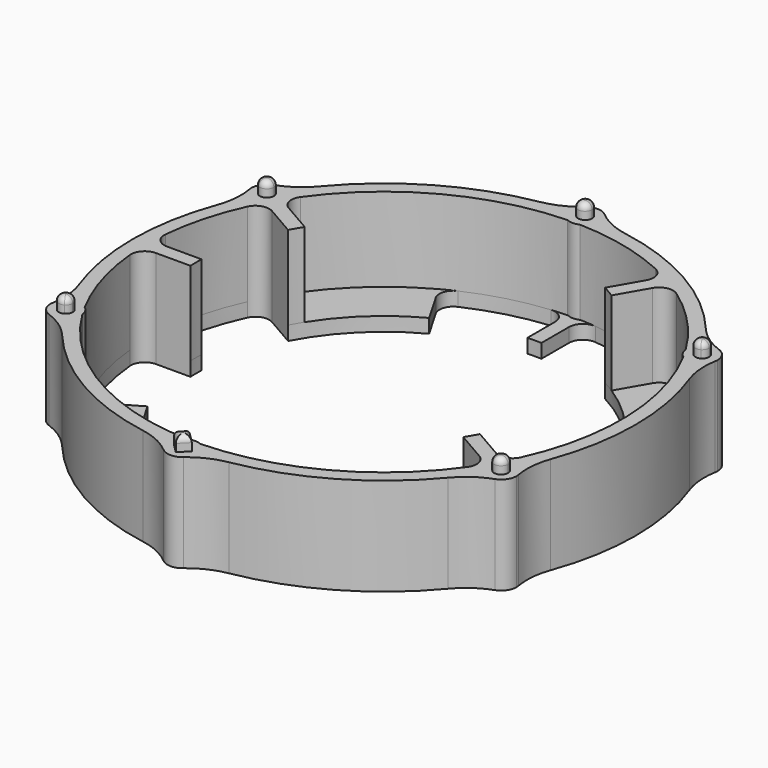
from build123d import *

# Parameters (mm, degrees)
F1_R         = 18
F1_R_2       = 17
F2_DEPTH     = 7
F3_DEPTH     = 7
F4_DEPTH     = 1
F6_DEPTH     = 7
F7_R         = 1
F8_R         = 5
F9_DEPTH     = 8
F10_R        = 0.44999
F11_DEPTH    = 1.8
F12_R        = 13.47
F13_DEPTH    = 1
F14_DEPTH    = 1
F15_T1_DEPTH = 3.7395798703
F15_T3_DEPTH = 1


# Not quite as in the source:
# - a fillet or chamfer that OpenCascade refuses, or shapes differently, is made with other operations: its cross-section is extruded or revolved along the edge and cut away or added
# - a fillet or chamfer is up to 0.001 mm smaller than in the source, because OpenCascade refuses the exact size


with BuildPart() as f2:
    # F1 (on Top) → F2 (new body)
    with BuildSketch(Plane.XY):
        Circle(F1_R)
        Circle(F1_R_2, mode=Mode.SUBTRACT)
    extrude(amount=F2_DEPTH)

    # F0 (on Top) → F3 (join)
    with BuildSketch(Plane.XY):
        with BuildLine():
            Line((-11.4073228059, 7.1633711619), (-14.4660626528, 8.9293354359))
            ThreePointArc((-14.4660626528, 8.9293354359), (-14.7224318643, 8.5), (-14.9660626528, 8.0633100321))
            Line((-14.9660626528, 8.0633100321), (-11.9073228059, 6.2973457581))
            ThreePointArc((-11.9073228059, 6.2973457581), (-11.665362189, 6.735), (-11.4073228059, 7.1633711619))
        make_face()
        with BuildLine():
            Line((7.1633711619, 11.4073228059), (8.9293354359, 14.4660626528))
            ThreePointArc((8.9293354359, 14.4660626528), (8.5, 14.7224318643), (8.0633100321, 14.9660626528))
            Line((8.0633100321, 14.9660626528), (6.2973457581, 11.9073228059))
            ThreePointArc((6.2973457581, 11.9073228059), (6.735, 11.665362189), (7.1633711619, 11.4073228059))
        make_face()
        with BuildLine():
            ThreePointArc((14.4660626528, -8.9293354359), (14.7224318643, -8.5), (14.9660626528, -8.0633100321))
            Line((14.9660626528, -8.0633100321), (11.9073228059, -6.2973457581))
            ThreePointArc((11.9073228059, -6.2973457581), (11.665362189, -6.735), (11.4073228059, -7.1633711619))
            Line((11.4073228059, -7.1633711619), (14.4660626528, -8.9293354359))
        make_face()
        with BuildLine():
            Line((-13.46071692, 0.5), (-16.992645468, 0.5))
            ThreePointArc((-16.992645468, 0.5), (-17, 0), (-16.992645468, -0.5))
            Line((-16.992645468, -0.5), (-13.46071692, -0.5))
            ThreePointArc((-13.46071692, -0.5), (-13.47, 0), (-13.46071692, 0.5))
        make_face()
    extrude(amount=F3_DEPTH)

    # F1 (on Top) → F4 (join)
    with BuildSketch(Plane.XY):
        Circle(F1_R)
        Circle(F1_R_2, mode=Mode.SUBTRACT)
        Circle(F1_R_2)
    extrude(amount=F4_DEPTH)

    # F5 (on Top) → F6 (join)
    with BuildSketch(Plane.XY):
        with BuildLine():
            ThreePointArc((-14.4884572681, 9), (-14.6275367743, 9.5353800561), (-15.0096060035, 9.935377578))
            ThreePointArc((-15.0096060035, 9.935377578), (-15.1731450826, 9.6837837802), (-15.3324673166, 9.4294987133))
            ThreePointArc((-15.3324673166, 9.4294987133), (-15.153718855, 9.2469868663), (-15.0884572681, 9))
            ThreePointArc((-15.0884572681, 9), (-15.3354561915, 8.5687338928), (-15.832419089, 8.5635568422))
            ThreePointArc((-15.832419089, 8.5635568422), (-15.9729752997, 8.2984372068), (-16.1090923805, 8.0310113108))
            ThreePointArc((-16.1090923805, 8.0310113108), (-15.0239657375, 8.0558870238), (-14.4884572681, 9))
        make_face()
        with BuildLine():
            ThreePointArc((-15.3324673166, 9.4294987133), (-15.1731450826, 9.6837837802), (-15.0096060035, 9.935377578))
            ThreePointArc((-15.0096060035, 9.935377578), (-16.5410852123, 9.55), (-16.1090923805, 8.0310113108))
            ThreePointArc((-16.1090923805, 8.0310113108), (-15.9729752997, 8.2984372068), (-15.832419089, 8.5635568422))
            ThreePointArc((-15.832419089, 8.5635568422), (-16.02146997, 9.25), (-15.3324673166, 9.4294987133))
        make_face()
        with BuildLine():
            ThreePointArc((-1.099486377, 17.9663888889), (0, 16.9), (1.099486377, 17.9663888889))
            ThreePointArc((1.099486377, 17.9663888889), (0.7998302171, 17.982220987), (0.4999517724, 17.9930555556))
            ThreePointArc((0.4999517724, 17.9930555556), (0, 17.5), (-0.4999517724, 17.9930555556))
            ThreePointArc((-0.4999517724, 17.9930555556), (-0.7998302171, 17.982220987), (-1.099486377, 17.9663888889))
        make_face()
        with BuildLine():
            ThreePointArc((0.4999517724, 17.9930555556), (0.7998302171, 17.982220987), (1.099486377, 17.9663888889))
            ThreePointArc((1.099486377, 17.9663888889), (1.0998715868, 17.9831924823), (1.1, 18))
            ThreePointArc((1.1, 18), (-0.0168075177, 19.0998715868), (-1.099486377, 17.9663888889))
            ThreePointArc((-1.099486377, 17.9663888889), (-0.7998302171, 17.982220987), (-0.4999517724, 17.9930555556))
            ThreePointArc((-0.4999517724, 17.9930555556), (-0.003472306, 18.4999879429), (0.5, 18))
            ThreePointArc((0.5, 18), (0.4999879429, 17.996527694), (0.4999517724, 17.9930555556))
        make_face()
        with BuildLine():
            ThreePointArc((15.832419089, 8.5635568422), (15.9729752997, 8.2984372068), (16.1090923805, 8.0310113108))
            ThreePointArc((16.1090923805, 8.0310113108), (16.5325702443, 8.4355084694), (16.6884572681, 9))
            ThreePointArc((16.6884572681, 9), (16.1238373242, 9.9609204939), (15.0096060035, 9.935377578))
            ThreePointArc((15.0096060035, 9.935377578), (15.1731450826, 9.6837837802), (15.3324673166, 9.4294987133))
            ThreePointArc((15.3324673166, 9.4294987133), (15.8354441344, 9.4347384132), (16.0884572681, 9))
            ThreePointArc((16.0884572681, 9), (16.0197233753, 8.7469989234), (15.832419089, 8.5635568422))
        make_face()
        with BuildLine():
            ThreePointArc((15.0096060035, 9.935377578), (14.635829324, 8.45), (16.1090923805, 8.0310113108))
            ThreePointArc((16.1090923805, 8.0310113108), (15.9729752997, 8.2984372068), (15.832419089, 8.5635568422))
            ThreePointArc((15.832419089, 8.5635568422), (15.1554445662, 8.75), (15.3324673166, 9.4294987133))
            ThreePointArc((15.3324673166, 9.4294987133), (15.1731450826, 9.6837837802), (15.0096060035, 9.935377578))
        make_face()
        with BuildLine():
            ThreePointArc((-15.3324673166, -9.4294987133), (-15.1731450826, -9.6837837802), (-15.0096060035, -9.935377578))
            ThreePointArc((-15.0096060035, -9.935377578), (-14.6275367743, -9.5353800561), (-14.4884572681, -9))
            ThreePointArc((-14.4884572681, -9), (-15.0239657375, -8.0558870238), (-16.1090923805, -8.0310113108))
            ThreePointArc((-16.1090923805, -8.0310113108), (-15.9729752997, -8.2984372068), (-15.832419089, -8.5635568422))
            ThreePointArc((-15.832419089, -8.5635568422), (-15.3354561915, -8.5687338928), (-15.0884572681, -9))
            ThreePointArc((-15.0884572681, -9), (-15.153718855, -9.2469868663), (-15.3324673166, -9.4294987133))
        make_face()
        with BuildLine():
            ThreePointArc((-16.1090923805, -8.0310113108), (-16.5410852123, -9.55), (-15.0096060035, -9.935377578))
            ThreePointArc((-15.0096060035, -9.935377578), (-15.1731450826, -9.6837837802), (-15.3324673166, -9.4294987133))
            ThreePointArc((-15.3324673166, -9.4294987133), (-16.02146997, -9.25), (-15.832419089, -8.5635568422))
            ThreePointArc((-15.832419089, -8.5635568422), (-15.9729752997, -8.2984372068), (-16.1090923805, -8.0310113108))
        make_face()
        with BuildLine():
            ThreePointArc((0.6255239257, -17.9891278226), (0.8625800837, -17.9793202207), (1.099486377, -17.9663888889))
            ThreePointArc((1.099486377, -17.9663888889), (0, -16.9), (-1.099486377, -17.9663888889))
            ThreePointArc((-1.099486377, -17.9663888889), (-0.8625800837, -17.9793202207), (-0.6255239257, -17.9891278226))
            Line((-0.6255239257, -17.9891278226), (0, -17.3636038969))
            Line((0, -17.3636038969), (0.6255239257, -17.9891278226))
        make_face()
        with BuildLine():
            ThreePointArc((1.1, -18), (1.0998715868, -17.9831924823), (1.099486377, -17.9663888889))
            ThreePointArc((1.099486377, -17.9663888889), (0.8625800837, -17.9793202207), (0.6255239257, -17.9891278226))
            Line((0.6255239257, -17.9891278226), (0.6363961031, -18))
            Line((0.6363961031, -18), (0, -18.6363961031))
            Line((0, -18.6363961031), (-0.6363961031, -18))
            Line((-0.6363961031, -18), (-0.6255239257, -17.9891278226))
            ThreePointArc((-0.6255239257, -17.9891278226), (-0.8625800837, -17.9793202207), (-1.099486377, -17.9663888889))
            ThreePointArc((-1.099486377, -17.9663888889), (-0.0168075177, -19.0998715868), (1.1, -18))
        make_face()
        with BuildLine():
            ThreePointArc((16.6884572681, -9), (16.5325702443, -8.4355084694), (16.1090923805, -8.0310113108))
            ThreePointArc((16.1090923805, -8.0310113108), (15.9729752997, -8.2984372068), (15.832419089, -8.5635568422))
            ThreePointArc((15.832419089, -8.5635568422), (16.0197233753, -8.7469989234), (16.0884572681, -9))
            ThreePointArc((16.0884572681, -9), (15.8354441344, -9.4347384132), (15.3324673166, -9.4294987133))
            ThreePointArc((15.3324673166, -9.4294987133), (15.1731450826, -9.6837837802), (15.0096060035, -9.935377578))
            ThreePointArc((15.0096060035, -9.935377578), (16.1238373242, -9.9609204939), (16.6884572681, -9))
        make_face()
        with BuildLine():
            ThreePointArc((15.832419089, -8.5635568422), (15.9729752997, -8.2984372068), (16.1090923805, -8.0310113108))
            ThreePointArc((16.1090923805, -8.0310113108), (14.635829324, -8.45), (15.0096060035, -9.935377578))
            ThreePointArc((15.0096060035, -9.935377578), (15.1731450826, -9.6837837802), (15.3324673166, -9.4294987133))
            ThreePointArc((15.3324673166, -9.4294987133), (15.1554445662, -8.75), (15.832419089, -8.5635568422))
        make_face()
        with BuildLine():
            ThreePointArc((-15.0884572681, 9), (-15.153718855, 9.2469868663), (-15.3324673166, 9.4294987133))
            ThreePointArc((-15.3324673166, 9.4294987133), (-15.5884572681, 9), (-15.832419089, 8.5635568422))
            ThreePointArc((-15.832419089, 8.5635568422), (-15.3354561915, 8.5687338928), (-15.0884572681, 9))
        make_face()
        with BuildLine():
            ThreePointArc((-15.832419089, 8.5635568422), (-15.5884572681, 9), (-15.3324673166, 9.4294987133))
            ThreePointArc((-15.3324673166, 9.4294987133), (-16.02146997, 9.25), (-15.832419089, 8.5635568422))
        make_face()
        with BuildLine():
            ThreePointArc((-0.4999517724, 17.9930555556), (0, 18), (0.4999517724, 17.9930555556))
            ThreePointArc((0.4999517724, 17.9930555556), (0.4999879429, 17.996527694), (0.5, 18))
            ThreePointArc((0.5, 18), (-0.003472306, 18.4999879429), (-0.4999517724, 17.9930555556))
        make_face()
        with BuildLine():
            ThreePointArc((-0.4999517724, 17.9930555556), (0, 17.5), (0.4999517724, 17.9930555556))
            ThreePointArc((0.4999517724, 17.9930555556), (0, 18), (-0.4999517724, 17.9930555556))
        make_face()
        with BuildLine():
            ThreePointArc((15.3324673166, 9.4294987133), (15.5884572681, 9), (15.832419089, 8.5635568422))
            ThreePointArc((15.832419089, 8.5635568422), (16.0197233753, 8.7469989234), (16.0884572681, 9))
            ThreePointArc((16.0884572681, 9), (15.8354441344, 9.4347384132), (15.3324673166, 9.4294987133))
        make_face()
        with BuildLine():
            ThreePointArc((15.3324673166, 9.4294987133), (15.1554445662, 8.75), (15.832419089, 8.5635568422))
            ThreePointArc((15.832419089, 8.5635568422), (15.5884572681, 9), (15.3324673166, 9.4294987133))
        make_face()
        with BuildLine():
            ThreePointArc((16.0884572681, -9), (16.0197233753, -8.7469989234), (15.832419089, -8.5635568422))
            ThreePointArc((15.832419089, -8.5635568422), (15.5884572681, -9), (15.3324673166, -9.4294987133))
            ThreePointArc((15.3324673166, -9.4294987133), (15.8354441344, -9.4347384132), (16.0884572681, -9))
        make_face()
        with BuildLine():
            ThreePointArc((15.3324673166, -9.4294987133), (15.5884572681, -9), (15.832419089, -8.5635568422))
            ThreePointArc((15.832419089, -8.5635568422), (15.1554445662, -8.75), (15.3324673166, -9.4294987133))
        make_face()
        with BuildLine():
            Line((0.6363961031, -18), (0.6255239257, -17.9891278226))
            ThreePointArc((0.6255239257, -17.9891278226), (0, -18), (-0.6255239257, -17.9891278226))
            Line((-0.6255239257, -17.9891278226), (-0.6363961031, -18))
            Line((-0.6363961031, -18), (0, -18.6363961031))
            Line((0, -18.6363961031), (0.6363961031, -18))
        make_face()
        with BuildLine():
            ThreePointArc((-15.832419089, -8.5635568422), (-16.02146997, -9.25), (-15.3324673166, -9.4294987133))
            ThreePointArc((-15.3324673166, -9.4294987133), (-15.5884572681, -9), (-15.832419089, -8.5635568422))
        make_face()
        with BuildLine():
            ThreePointArc((-15.832419089, -8.5635568422), (-15.5884572681, -9), (-15.3324673166, -9.4294987133))
            ThreePointArc((-15.3324673166, -9.4294987133), (-15.153718855, -9.2469868663), (-15.0884572681, -9))
            ThreePointArc((-15.0884572681, -9), (-15.3354561915, -8.5687338928), (-15.832419089, -8.5635568422))
        make_face()
        with BuildLine():
            ThreePointArc((-0.6255239257, -17.9891278226), (0, -18), (0.6255239257, -17.9891278226))
            Line((0.6255239257, -17.9891278226), (0, -17.3636038969))
            Line((0, -17.3636038969), (-0.6255239257, -17.9891278226))
        make_face()
    extrude(amount=F6_DEPTH)

    # F7
    f7_edges = [f2.edges().sort_by_distance(p)[0] for p in [
        (8.06331, 14.966063, 4),
        (-16.992645, 0.5, 4),
        (14.966063, -8.06331, 4),
        (-16.992645, -0.5, 4),
        (-14.966063, 8.06331, 4),
        (-14.466063, 8.929335, 4),
        (8.929335, 14.466063, 4),
        (14.466063, -8.929335, 4),
    ]]
    fillet(f7_edges, radius=F7_R)

    # F8 (call 1 of 12: OpenCascade refuses the feature's edges together)
    f8_edges = [f2.edges().sort_by_distance(p)[0] for p in [
        (-16.109092, 8.031011, 3.5),
    ]]
    fillet(f8_edges, radius=F8_R)

    # F8#2 (call 2 of 12)
    f8_2_edges = [f2.edges().sort_by_distance(p)[0] for p in [
        (-15.009606, 9.935378, 3.5),
    ]]
    fillet(f8_2_edges, radius=F8_R)

    # F8#3 (call 3 of 12)
    f8_3_edges = [f2.edges().sort_by_distance(p)[0] for p in [
        (-1.099486, 17.966389, 3.5),
    ]]
    fillet(f8_3_edges, radius=F8_R)

    # F8#4 (call 4 of 12)
    f8_4_edges = [f2.edges().sort_by_distance(p)[0] for p in [
        (1.099486, 17.966389, 3.5),
    ]]
    fillet(f8_4_edges, radius=F8_R)

    # F8#5 (call 5 of 12)
    f8_5_edges = [f2.edges().sort_by_distance(p)[0] for p in [
        (-15.009606, -9.935378, 3.5),
    ]]
    fillet(f8_5_edges, radius=F8_R)

    # F8#6 (call 6 of 12)
    f8_6_edges = [f2.edges().sort_by_distance(p)[0] for p in [
        (-16.109092, -8.031011, 3.5),
    ]]
    fillet(f8_6_edges, radius=F8_R)

    # F8#7 (call 7 of 12)
    f8_7_edges = [f2.edges().sort_by_distance(p)[0] for p in [
        (1.099486, -17.966389, 3.5),
    ]]
    fillet(f8_7_edges, radius=F8_R)

    # F8#8 (call 8 of 12)
    f8_8_edges = [f2.edges().sort_by_distance(p)[0] for p in [
        (-1.099486, -17.966389, 3.5),
    ]]
    fillet(f8_8_edges, radius=F8_R)

    # F8#10 (call 9 of 12)
    f8_10_edges = [f2.edges().sort_by_distance(p)[0] for p in [
        (15.009606, -9.935378, 3.5),
    ]]
    fillet(f8_10_edges, radius=F8_R)

    # F8#11 (call 10 of 12)
    f8_11_edges = [f2.edges().sort_by_distance(p)[0] for p in [
        (16.109092, 8.031011, 3.5),
    ]]
    fillet(f8_11_edges, radius=F8_R)

    # F8#12 (call 11 of 12)
    f8_12_edges = [f2.edges().sort_by_distance(p)[0] for p in [
        (15.009606, 9.935378, 3.5),
    ]]
    fillet(f8_12_edges, radius=F8_R)

    # F8#9 (call 12 of 12)
    f8_9_edges = [f2.edges().sort_by_distance(p)[0] for p in [
        (16.109092, -8.031011, 3.5),
    ]]
    fillet(f8_9_edges, radius=F8_R)

    # F5 (on Top) → F9 (join)
    with BuildSketch(Plane.XY):
        with BuildLine():
            ThreePointArc((-15.832419089, 8.5635568422), (-15.5884572681, 9), (-15.3324673166, 9.4294987133))
            ThreePointArc((-15.3324673166, 9.4294987133), (-16.02146997, 9.25), (-15.832419089, 8.5635568422))
        make_face()
        with BuildLine():
            ThreePointArc((-15.0884572681, 9), (-15.153718855, 9.2469868663), (-15.3324673166, 9.4294987133))
            ThreePointArc((-15.3324673166, 9.4294987133), (-15.5884572681, 9), (-15.832419089, 8.5635568422))
            ThreePointArc((-15.832419089, 8.5635568422), (-15.3354561915, 8.5687338928), (-15.0884572681, 9))
        make_face()
        with BuildLine():
            ThreePointArc((-0.4999517724, 17.9930555556), (0, 18), (0.4999517724, 17.9930555556))
            ThreePointArc((0.4999517724, 17.9930555556), (0.4999879429, 17.996527694), (0.5, 18))
            ThreePointArc((0.5, 18), (-0.003472306, 18.4999879429), (-0.4999517724, 17.9930555556))
        make_face()
        with BuildLine():
            ThreePointArc((-0.4999517724, 17.9930555556), (0, 17.5), (0.4999517724, 17.9930555556))
            ThreePointArc((0.4999517724, 17.9930555556), (0, 18), (-0.4999517724, 17.9930555556))
        make_face()
        with BuildLine():
            ThreePointArc((15.3324673166, 9.4294987133), (15.1554445662, 8.75), (15.832419089, 8.5635568422))
            ThreePointArc((15.832419089, 8.5635568422), (15.5884572681, 9), (15.3324673166, 9.4294987133))
        make_face()
        with BuildLine():
            ThreePointArc((15.3324673166, 9.4294987133), (15.5884572681, 9), (15.832419089, 8.5635568422))
            ThreePointArc((15.832419089, 8.5635568422), (16.0197233753, 8.7469989234), (16.0884572681, 9))
            ThreePointArc((16.0884572681, 9), (15.8354441344, 9.4347384132), (15.3324673166, 9.4294987133))
        make_face()
        with BuildLine():
            ThreePointArc((15.3324673166, -9.4294987133), (15.5884572681, -9), (15.832419089, -8.5635568422))
            ThreePointArc((15.832419089, -8.5635568422), (15.1554445662, -8.75), (15.3324673166, -9.4294987133))
        make_face()
        with BuildLine():
            ThreePointArc((16.0884572681, -9), (16.0197233753, -8.7469989234), (15.832419089, -8.5635568422))
            ThreePointArc((15.832419089, -8.5635568422), (15.5884572681, -9), (15.3324673166, -9.4294987133))
            ThreePointArc((15.3324673166, -9.4294987133), (15.8354441344, -9.4347384132), (16.0884572681, -9))
        make_face()
        with BuildLine():
            Line((0.6363961031, -18), (0.6255239257, -17.9891278226))
            ThreePointArc((0.6255239257, -17.9891278226), (0, -18), (-0.6255239257, -17.9891278226))
            Line((-0.6255239257, -17.9891278226), (-0.6363961031, -18))
            Line((-0.6363961031, -18), (0, -18.6363961031))
            Line((0, -18.6363961031), (0.6363961031, -18))
        make_face()
        with BuildLine():
            ThreePointArc((-0.6255239257, -17.9891278226), (0, -18), (0.6255239257, -17.9891278226))
            Line((0.6255239257, -17.9891278226), (0, -17.3636038969))
            Line((0, -17.3636038969), (-0.6255239257, -17.9891278226))
        make_face()
        with BuildLine():
            ThreePointArc((-15.832419089, -8.5635568422), (-16.02146997, -9.25), (-15.3324673166, -9.4294987133))
            ThreePointArc((-15.3324673166, -9.4294987133), (-15.5884572681, -9), (-15.832419089, -8.5635568422))
        make_face()
        with BuildLine():
            ThreePointArc((-15.832419089, -8.5635568422), (-15.5884572681, -9), (-15.3324673166, -9.4294987133))
            ThreePointArc((-15.3324673166, -9.4294987133), (-15.153718855, -9.2469868663), (-15.0884572681, -9))
            ThreePointArc((-15.0884572681, -9), (-15.3354561915, -8.5687338928), (-15.832419089, -8.5635568422))
        make_face()
    extrude(amount=F9_DEPTH)

    # F10 (radius 0.45 in the source; OpenCascade refuses exactly that, so slightly less here)
    f10_edges = [f2.edges().sort_by_distance(p)[0] for p in [
        (-15.844447, -8.570501, 8),
        (-15.344495, 9.436443, 8),
        (0.499952, 18.006944, 8),
        (15.344495, 9.436443, 8),
        (15.844447, -8.570501, 8),
        (0.318198, -17.681802, 8),
        (-0.318198, -18.318198, 8),
        (0.318198, -18.318198, 8),
        (-0.318198, -17.681802, 8),
    ]]
    fillet(f10_edges, radius=F10_R)

    # F5 (on Top) → F11 (cut)
    with BuildSketch(Plane.XY):
        with BuildLine():
            ThreePointArc((-15.832419089, -8.5635568422), (-16.02146997, -9.25), (-15.3324673166, -9.4294987133))
            ThreePointArc((-15.3324673166, -9.4294987133), (-15.5884572681, -9), (-15.832419089, -8.5635568422))
        make_face()
        with BuildLine():
            ThreePointArc((-15.832419089, -8.5635568422), (-15.5884572681, -9), (-15.3324673166, -9.4294987133))
            ThreePointArc((-15.3324673166, -9.4294987133), (-15.153718855, -9.2469868663), (-15.0884572681, -9))
            ThreePointArc((-15.0884572681, -9), (-15.3354561915, -8.5687338928), (-15.832419089, -8.5635568422))
        make_face()
        with BuildLine():
            Line((0.6363961031, -18), (0.6255239257, -17.9891278226))
            ThreePointArc((0.6255239257, -17.9891278226), (0, -18), (-0.6255239257, -17.9891278226))
            Line((-0.6255239257, -17.9891278226), (-0.6363961031, -18))
            Line((-0.6363961031, -18), (0, -18.6363961031))
            Line((0, -18.6363961031), (0.6363961031, -18))
        make_face()
        with BuildLine():
            ThreePointArc((-0.6255239257, -17.9891278226), (0, -18), (0.6255239257, -17.9891278226))
            Line((0.6255239257, -17.9891278226), (0, -17.3636038969))
            Line((0, -17.3636038969), (-0.6255239257, -17.9891278226))
        make_face()
        with BuildLine():
            ThreePointArc((15.3324673166, -9.4294987133), (15.5884572681, -9), (15.832419089, -8.5635568422))
            ThreePointArc((15.832419089, -8.5635568422), (15.1554445662, -8.75), (15.3324673166, -9.4294987133))
        make_face()
        with BuildLine():
            ThreePointArc((16.0884572681, -9), (16.0197233753, -8.7469989234), (15.832419089, -8.5635568422))
            ThreePointArc((15.832419089, -8.5635568422), (15.5884572681, -9), (15.3324673166, -9.4294987133))
            ThreePointArc((15.3324673166, -9.4294987133), (15.8354441344, -9.4347384132), (16.0884572681, -9))
        make_face()
        with BuildLine():
            ThreePointArc((15.3324673166, 9.4294987133), (15.1554445662, 8.75), (15.832419089, 8.5635568422))
            ThreePointArc((15.832419089, 8.5635568422), (15.5884572681, 9), (15.3324673166, 9.4294987133))
        make_face()
        with BuildLine():
            ThreePointArc((15.3324673166, 9.4294987133), (15.5884572681, 9), (15.832419089, 8.5635568422))
            ThreePointArc((15.832419089, 8.5635568422), (16.0197233753, 8.7469989234), (16.0884572681, 9))
            ThreePointArc((16.0884572681, 9), (15.8354441344, 9.4347384132), (15.3324673166, 9.4294987133))
        make_face()
        with BuildLine():
            ThreePointArc((-0.4999517724, 17.9930555556), (0, 17.5), (0.4999517724, 17.9930555556))
            ThreePointArc((0.4999517724, 17.9930555556), (0, 18), (-0.4999517724, 17.9930555556))
        make_face()
        with BuildLine():
            ThreePointArc((-0.4999517724, 17.9930555556), (0, 18), (0.4999517724, 17.9930555556))
            ThreePointArc((0.4999517724, 17.9930555556), (0.4999879429, 17.996527694), (0.5, 18))
            ThreePointArc((0.5, 18), (-0.003472306, 18.4999879429), (-0.4999517724, 17.9930555556))
        make_face()
        with BuildLine():
            ThreePointArc((-15.832419089, 8.5635568422), (-15.5884572681, 9), (-15.3324673166, 9.4294987133))
            ThreePointArc((-15.3324673166, 9.4294987133), (-16.02146997, 9.25), (-15.832419089, 8.5635568422))
        make_face()
        with BuildLine():
            ThreePointArc((-15.0884572681, 9), (-15.153718855, 9.2469868663), (-15.3324673166, 9.4294987133))
            ThreePointArc((-15.3324673166, 9.4294987133), (-15.5884572681, 9), (-15.832419089, 8.5635568422))
            ThreePointArc((-15.832419089, 8.5635568422), (-15.3354561915, 8.5687338928), (-15.0884572681, 9))
        make_face()
    extrude(amount=F11_DEPTH, mode=Mode.SUBTRACT)

    # F12 (on Top) → F13 (cut)
    with BuildSketch(Plane.XY):
        Circle(F12_R)
    extrude(amount=F13_DEPTH, mode=Mode.SUBTRACT)

    # F0 (on Top) → F14 (cut)
    with BuildSketch(Plane.XY):
        with BuildLine():
            ThreePointArc((0.5, -16.992645468), (4.3999237667, -16.4207390469), (8.0633100321, -14.9660626528))
            Line((8.0633100321, -14.9660626528), (6.2973457581, -11.9073228059))
            ThreePointArc((6.2973457581, -11.9073228059), (3.4862925375, -13.0110208801), (0.5, -13.46071692))
            Line((0.5, -13.46071692), (0.5, -16.992645468))
        make_face()
        with BuildLine():
            ThreePointArc((8.9293354359, -14.4660626528), (12.0208152802, -12.0208152802), (14.4660626528, -8.9293354359))
            Line((14.4660626528, -8.9293354359), (11.4073228059, -7.1633711619))
            ThreePointArc((11.4073228059, -7.1633711619), (9.5247283426, -9.5247283426), (7.1633711619, -11.4073228059))
            Line((7.1633711619, -11.4073228059), (8.9293354359, -14.4660626528))
        make_face()
        with BuildLine():
            ThreePointArc((14.9660626528, -8.0633100321), (16.4207390469, -4.3999237667), (16.992645468, -0.5))
            Line((16.992645468, -0.5), (13.46071692, -0.5))
            ThreePointArc((13.46071692, -0.5), (13.0110208801, -3.4862925375), (11.9073228059, -6.2973457581))
            Line((11.9073228059, -6.2973457581), (14.9660626528, -8.0633100321))
        make_face()
        with BuildLine():
            Line((6.2973457581, 11.9073228059), (8.0633100321, 14.9660626528))
            ThreePointArc((8.0633100321, 14.9660626528), (4.3999237667, 16.4207390469), (0.5, 16.992645468))
            Line((0.5, 16.992645468), (0.5, 13.46071692))
            ThreePointArc((0.5, 13.46071692), (3.4862925375, 13.0110208801), (6.2973457581, 11.9073228059))
        make_face()
        with BuildLine():
            Line((-0.5, 13.46071692), (-0.5, 16.992645468))
            ThreePointArc((-0.5, 16.992645468), (-4.3999237667, 16.4207390469), (-8.0633100321, 14.9660626528))
            Line((-8.0633100321, 14.9660626528), (-6.2973457581, 11.9073228059))
            ThreePointArc((-6.2973457581, 11.9073228059), (-3.4862925375, 13.0110208801), (-0.5, 13.46071692))
        make_face()
        with BuildLine():
            Line((-11.9073228059, 6.2973457581), (-14.9660626528, 8.0633100321))
            ThreePointArc((-14.9660626528, 8.0633100321), (-16.4207390469, 4.3999237667), (-16.992645468, 0.5))
            Line((-16.992645468, 0.5), (-13.46071692, 0.5))
            ThreePointArc((-13.46071692, 0.5), (-13.0110208801, 3.4862925375), (-11.9073228059, 6.2973457581))
        make_face()
        with BuildLine():
            ThreePointArc((-16.992645468, -0.5), (-16.4207390469, -4.3999237667), (-14.9660626528, -8.0633100321))
            Line((-14.9660626528, -8.0633100321), (-11.9073228059, -6.2973457581))
            ThreePointArc((-11.9073228059, -6.2973457581), (-13.0110208801, -3.4862925375), (-13.46071692, -0.5))
            Line((-13.46071692, -0.5), (-16.992645468, -0.5))
        make_face()
    extrude(amount=F14_DEPTH, mode=Mode.SUBTRACT)

    # F15: fillet of radius 1 on 14 edges, made by hand

    # F15_s2 → F15_t1 (join)
    with BuildSketch(Plane.XY):
        with BuildLine():
            ThreePointArc((-16.9251280922, -1.59375), (-16.669042295, -0.8268543991), (-15.9295323221, -0.5))
            Line((-15.9295323221, -0.5), (-16.992645468, -0.5))
            ThreePointArc((-16.992645468, -0.5), (-16.9677020567, -1.0474191685), (-16.9251280922, -1.59375))
        make_face()
        with BuildLine():
            ThreePointArc((-15.4544658902, 7.0823360588), (-14.8492412837, 7.6184442326), (-14.0453796613, 7.5317534591))
            Line((-14.0453796613, 7.5317534591), (-14.9660626528, 8.0633100321))
            ThreePointArc((-14.9660626528, 8.0633100321), (-15.2181706092, 7.57675942), (-15.4544658902, 7.0823360588))
        make_face()
        with BuildLine():
            ThreePointArc((-15.9295323221, 0.5), (-16.669042295, 0.8268543991), (-16.9251280922, 1.59375))
            ThreePointArc((-16.9251280922, 1.59375), (-16.9677020567, 1.0474191685), (-16.992645468, 0.5))
            Line((-16.992645468, 0.5), (-15.9295323221, 0.5))
        make_face()
        with BuildLine():
            ThreePointArc((14.0453796613, -7.5317534591), (14.8492412838, -7.6184442326), (15.4544658902, -7.0823360588))
            ThreePointArc((15.4544658902, -7.0823360588), (15.2181706092, -7.57675942), (14.9660626528, -8.0633100321))
            Line((14.9660626528, -8.0633100321), (14.0453796613, -7.5317534591))
        make_face()
        with BuildLine():
            ThreePointArc((7.5317534591, 14.0453796613), (7.6184442326, 14.8492412838), (7.0823360588, 15.4544658902))
            ThreePointArc((7.0823360588, 15.4544658902), (7.57675942, 15.2181706092), (8.0633100321, 14.9660626528))
            Line((8.0633100321, 14.9660626528), (7.5317534591, 14.0453796613))
        make_face()
        with BuildLine():
            ThreePointArc((13.5453796613, -8.3977788629), (14.0223868846, -9.0505980623), (13.8607158902, -9.8427920334))
            ThreePointArc((13.8607158902, -9.8427920334), (14.1707514407, -9.3909426367), (14.4660626528, -8.9293354359))
            Line((14.4660626528, -8.9293354359), (13.5453796613, -8.3977788629))
        make_face()
    extrude(amount=F15_T1_DEPTH)

    # F15_s4 → F15_t3 (join)
    with BuildSketch(Plane.XY):
        with BuildLine():
            ThreePointArc((1.59375, 16.9251280922), (0.8268543991, 16.669042295), (0.5, 15.9295323221))
            Line((0.5, 15.9295323221), (0.5, 16.992645468))
            ThreePointArc((0.5, 16.992645468), (1.0474191685, 16.9677020567), (1.59375, 16.9251280922))
        make_face()
        with BuildLine():
            ThreePointArc((-7.0823360588, 15.4544658902), (-7.6184442326, 14.8492412837), (-7.5317534591, 14.0453796613))
            Line((-7.5317534591, 14.0453796613), (-8.0633100321, 14.9660626528))
            ThreePointArc((-8.0633100321, 14.9660626528), (-7.57675942, 15.2181706092), (-7.0823360588, 15.4544658902))
        make_face()
        with BuildLine():
            ThreePointArc((-15.4544658902, -7.0823360588), (-14.8492412837, -7.6184442326), (-14.0453796613, -7.5317534591))
            Line((-14.0453796613, -7.5317534591), (-14.9660626528, -8.0633100321))
            ThreePointArc((-14.9660626528, -8.0633100321), (-15.2181706092, -7.57675942), (-15.4544658902, -7.0823360588))
        make_face()
        with BuildLine():
            ThreePointArc((1.59375, -16.9251280922), (0.8268543991, -16.669042295), (0.5, -15.9295323221))
            Line((0.5, -15.9295323221), (0.5, -16.992645468))
            ThreePointArc((0.5, -16.992645468), (1.0474191685, -16.9677020567), (1.59375, -16.9251280922))
        make_face()
        with BuildLine():
            ThreePointArc((9.8427920334, -13.8607158902), (9.0505980623, -14.0223868846), (8.3977788629, -13.5453796613))
            Line((8.3977788629, -13.5453796613), (8.9293354359, -14.4660626528))
            ThreePointArc((8.9293354359, -14.4660626528), (9.3909426367, -14.1707514407), (9.8427920334, -13.8607158902))
        make_face()
        with BuildLine():
            ThreePointArc((16.9251280922, -1.59375), (16.669042295, -0.8268543991), (15.9295323221, -0.5))
            Line((15.9295323221, -0.5), (16.992645468, -0.5))
            ThreePointArc((16.992645468, -0.5), (16.9677020567, -1.0474191685), (16.9251280922, -1.59375))
        make_face()
        with BuildLine():
            ThreePointArc((-1.59375, 16.9251280922), (-0.8268543991, 16.669042295), (-0.5, 15.9295323221))
            Line((-0.5, 15.9295323221), (-0.5, 16.992645468))
            ThreePointArc((-0.5, 16.992645468), (-1.0474191685, 16.9677020567), (-1.59375, 16.9251280922))
        make_face()
        with BuildLine():
            ThreePointArc((7.0823360588, -15.4544658902), (7.6184442326, -14.8492412837), (7.5317534591, -14.0453796613))
            Line((7.5317534591, -14.0453796613), (8.0633100321, -14.9660626528))
            ThreePointArc((8.0633100321, -14.9660626528), (7.57675942, -15.2181706092), (7.0823360588, -15.4544658902))
        make_face()
    extrude(amount=F15_T3_DEPTH)


solid = f2.part
